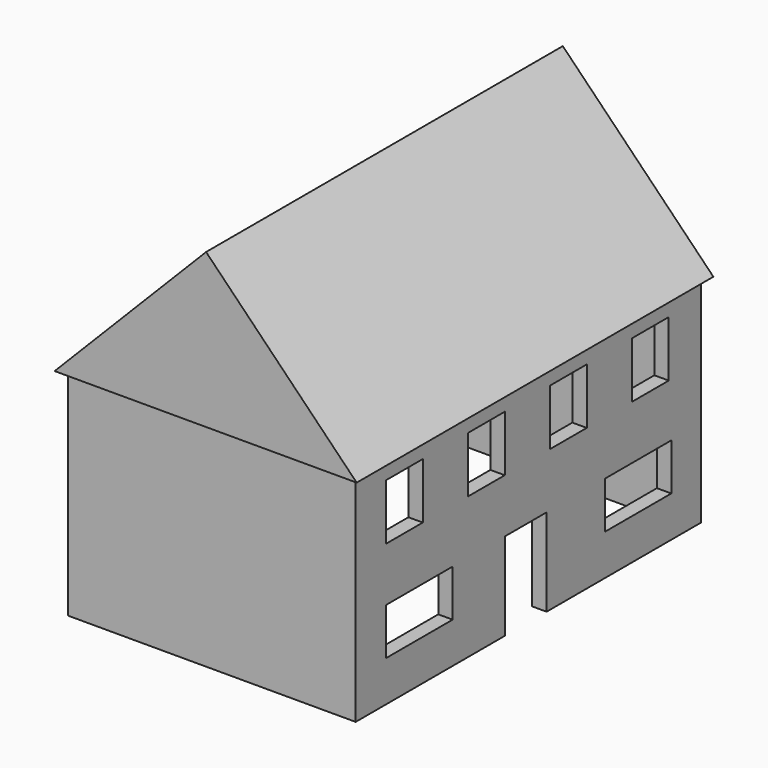
from build123d import *

# Parameters (mm, degrees)
F0_W          = 50.8
F0_H          = 38.1
F2_DEPTH      = 38.1
F2_DEPTH_BACK = 38.1
F3_DEPTH      = 39.37
F3_DEPTH_BACK = 39.37
F4_T          = -2.54
F6_W          = 9.1468244791
F6_H          = 15.4547751881
F6_W_2        = 8.080781489
F6_H_2        = 9.8759858869
F6_W_3        = 14.6728920285
F6_H_3        = 8.2574296976
F7_DEPTH      = 2.54


# Not quite as in the source:
# - the program builds the solid bodies; features that only make, move or delete a surface that nothing else refers to are left out


with BuildPart() as f2:
    # F0 (on Front) → F2 (new body, two sides)
    with BuildSketch(Plane.XZ) as f2_sk:
        with Locations((0, 19.05)):
            Rectangle(F0_W, F0_H)
    extrude(amount=F2_DEPTH)
    extrude(f2_sk.sketch, amount=-F2_DEPTH_BACK)

    # F1 (on Front) → F3 (join, two sides)
    with BuildSketch(Plane.XZ) as f3_sk:
        Polygon((0, 65.3146550722), (-26.7503901826, 38.1), (26.5896098174, 38.1), align=None)
    extrude(amount=F3_DEPTH)
    extrude(f3_sk.sketch, amount=-F3_DEPTH_BACK)

    # F4
    f4_openings = [f2.faces().sort_by_distance(p)[0] for p in [
        (0, 0, 0),
    ]]
    offset(amount=F4_T, openings=f4_openings, kind=Kind.INTERSECTION)

    # F6 (on offset) → F7 (cut)
    with BuildSketch(Plane.YZ.offset(25.4)):
        with Locations((-0.5318810698, 7.7273875941)):
            Rectangle(F6_W, F6_H)
        with Locations((-27.3286092555, 29.9121104646)):
            Rectangle(F6_W_2, F6_H_2)
        with Locations((-9.2311092555, 29.9121104646)):
            Rectangle(F6_W_2, F6_H_2)
        with Locations((8.8663907445, 29.9121104646)):
            Rectangle(F6_W_2, F6_H_2)
        with Locations((26.9638907445, 29.9121104646)):
            Rectangle(F6_W_2, F6_H_2)
        with Locations((24.2274460142, 11.3260603393)):
            Rectangle(F6_W_3, F6_H_3)
        with Locations((-24.0325539858, 11.3260603393)):
            Rectangle(F6_W_3, F6_H_3)
    extrude(amount=-F7_DEPTH, mode=Mode.SUBTRACT)


solid = f2.part
